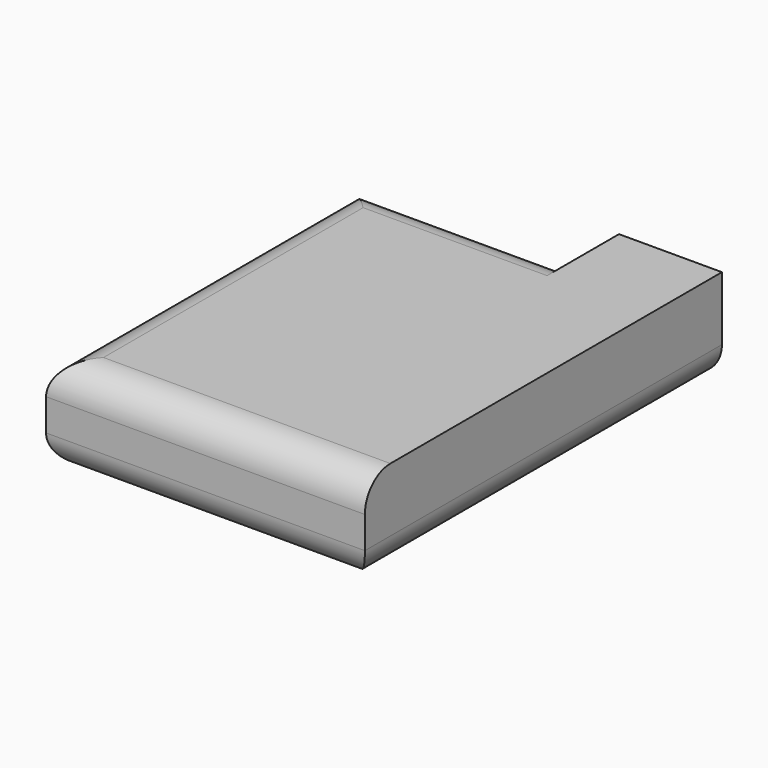
from build123d import *

# Parameters (mm, degrees)
F1_DEPTH    = 15
F2_W        = 46.8627084047
F2_H        = 56.3212386332
F3_DEPTH    = 13.30162
F4_W        = 13.7536320835
F4_H        = 12.7884671092
F5_DEPTH    = 13.81799
F6_T1_DEPTH = 75
F6_T3_DEPTH = 85.9022176913
F6_T5_DEPTH = 46.3573584799
F6_T7_DEPTH = 95


# Not quite as in the source:
# - a fillet or chamfer that OpenCascade refuses, or shapes differently, is made with other operations: its cross-section is extruded or revolved along the edge and cut away or added


with BuildPart() as f1:
    # F0 (on Top) → F1 (new body)
    with BuildSketch(Plane.XY):
        Polygon((-57.3696343694, 65.8665671945), (-57.3696343694, 4.9643495032), (-7.3696343694, 4.9643495032), (-7.3696343694, 74.9643495032), (-23.5122758895, 74.9643495032), (-23.5122758895, 65.8665671945), align=None)
    extrude(amount=F1_DEPTH)

    # F2 (on Top) → F3 (cut)
    with BuildSketch(Plane.XY):
        with Locations((-32.3047889397, 34.9865604658)):
            Rectangle(F2_W, F2_H)
    extrude(amount=F3_DEPTH, mode=Mode.SUBTRACT)

    # F4 (on Top) → F5 (cut)
    with BuildSketch(Plane.XY):
        with Locations((-15.8223016188, 69.8727704585)):
            Rectangle(F4_W, F4_H)
    extrude(amount=F5_DEPTH, mode=Mode.SUBTRACT)

    # F6: fillet of radius 5 on 6 edges, made by hand

    # F6_s2 → F6_t1 (cut)
    with BuildSketch(Plane.YZ.offset(-69.8696343694)):
        with BuildLine():
            ThreePointArc((4.9643495032, 10), (6.4288155972, 13.5355339059), (9.9643495032, 15))
            Line((9.9643495032, 15), (4.9643495032, 15))
            Line((4.9643495032, 15), (4.9643495032, 10))
        make_face()
        with BuildLine():
            ThreePointArc((4.9643495032, 5), (6.4288155972, 1.4644660941), (9.9643495032, 0))
            Line((9.9643495032, 0), (4.9643495032, 0))
            Line((4.9643495032, 0), (4.9643495032, 5))
        make_face()
    extrude(amount=F6_T1_DEPTH, mode=Mode.SUBTRACT)

    # F6_s4 → F6_t3 (cut)
    with BuildSketch(Plane.XZ.offset(-78.3665671945)):
        with BuildLine():
            ThreePointArc((-57.3696343694, 10), (-55.9051682753, 13.5355339059), (-52.3696343694, 15))
            Line((-52.3696343694, 15), (-57.3696343694, 15))
            Line((-57.3696343694, 15), (-57.3696343694, 10))
        make_face()
        with BuildLine():
            ThreePointArc((-57.3696343694, 5), (-55.9051682753, 1.4644660941), (-52.3696343694, 0))
            Line((-52.3696343694, 0), (-57.3696343694, 0))
            Line((-57.3696343694, 0), (-57.3696343694, 5))
        make_face()
    extrude(amount=F6_T3_DEPTH, mode=Mode.SUBTRACT)

    # F6_s6 → F6_t5 (cut)
    with BuildSketch(Plane.YZ.offset(-69.8696343694)):
        with BuildLine():
            ThreePointArc((65.8665671945, 10), (64.4021011004, 13.5355339059), (60.8665671945, 15))
            Line((60.8665671945, 15), (65.8665671945, 15))
            Line((65.8665671945, 15), (65.8665671945, 10))
        make_face()
    extrude(amount=F6_T5_DEPTH, mode=Mode.SUBTRACT)

    # F6_s8 → F6_t7 (cut)
    with BuildSketch(Plane.XZ.offset(-87.4643495032)):
        with BuildLine():
            ThreePointArc((-12.3696343694, 0), (-8.8341004635, 1.4644660941), (-7.3696343694, 5))
            Line((-7.3696343694, 5), (-7.3696343694, 0))
            Line((-7.3696343694, 0), (-12.3696343694, 0))
        make_face()
    extrude(amount=F6_T7_DEPTH, mode=Mode.SUBTRACT)


solid = f1.part
